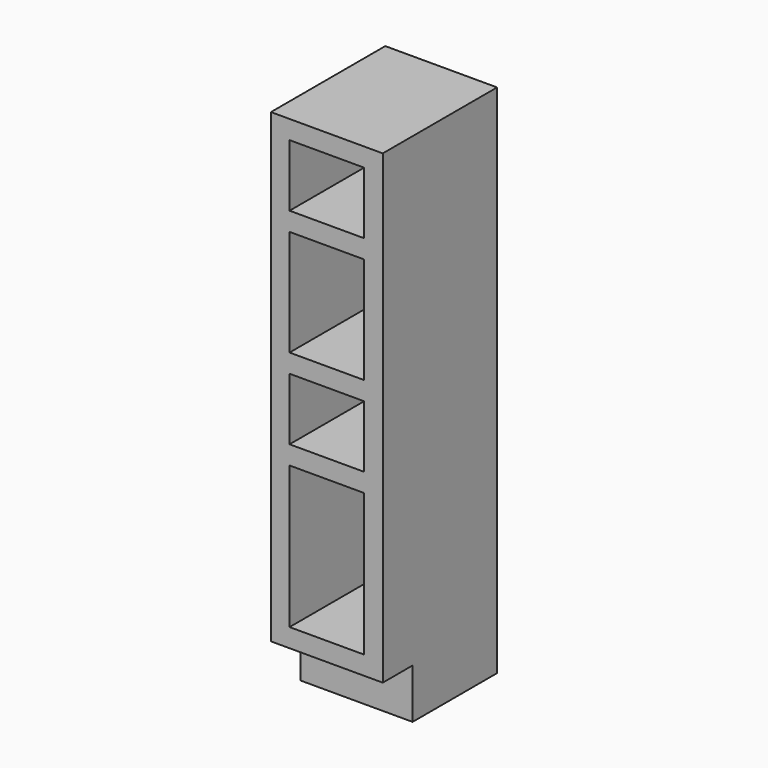
from build123d import *

# Parameters (mm, degrees)
F1_DEPTH = 228.6
F2_W     = 152.4
F2_H     = 127
F2_H_2   = 217.1721715927
F2_H_3   = 290.8278284073
F3_DEPTH = 279.4


# Not quite as in the source:
# - a feature names something its author has since deleted; it is built from what else it names


with BuildPart() as f1:
    # F0 (on Right) → F1 (new body)
    with BuildSketch(Plane.YZ):
        Polygon((-215.9, 0), (0, 0), (0, 1054.1), (-292.1, 1054.1), (-292.1, 101.6), (-215.9, 101.6), align=None)
    extrude(amount=F1_DEPTH)

    # F2 (on face) → F3 (cut)
    with BuildSketch(Plane.XZ.offset(292.1)):
        with Locations((114.3, 952.5)):
            Rectangle(F2_W, F2_H)
        with Locations((114.3, 742.3139142036)):
            Rectangle(F2_W, F2_H_2)
        with Locations((114.3, 532.1278284073)):
            Rectangle(F2_W, F2_H)
        with Locations((114.3, 285.1139142036)):
            Rectangle(F2_W, F2_H_3)
    extrude(amount=-F3_DEPTH, mode=Mode.SUBTRACT)


solid = f1.part
